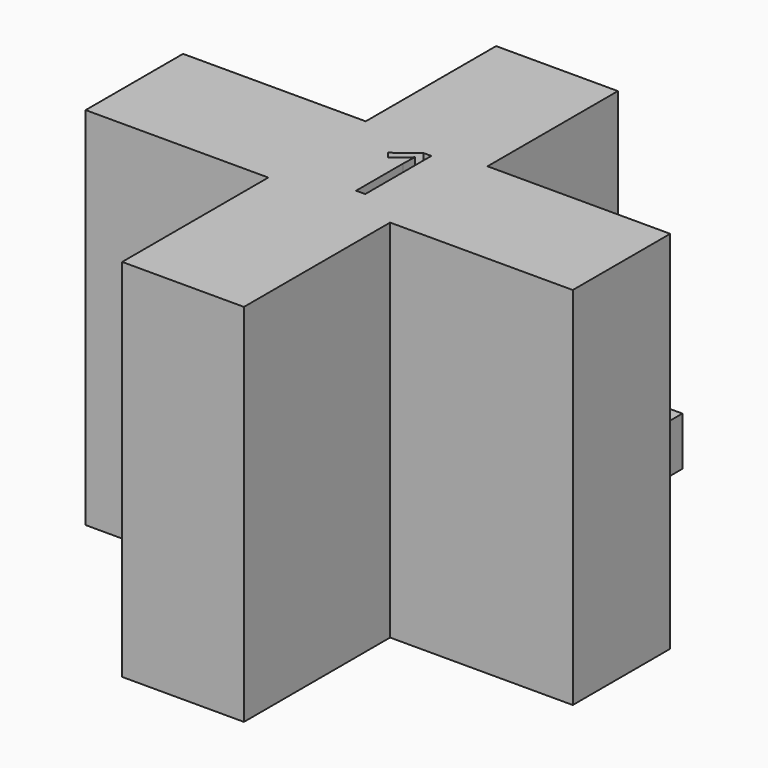
from build123d import *

# Parameters (mm, degrees)
F0_W         = 12.7
F0_H         = 57.15
F1_DEPTH     = 5.08
F2_W         = 50.8
F2_H         = 12.7
F3_DEPTH     = 38.1
F4_W         = 12.7
F4_H         = 48.7413735385
F5_DEPTH     = 33.02
F6_TEXT_SIZE = 12.0747026004
F7_DEPTH     = 2.54


# Not quite as in the source:
# - Text() gives the source's letters only with a copy of the font that has no kerning and outlines rounded to 1/6400 em; it was checked with that copy


with BuildPart() as f1:
    # F0 (on Top) → F1 (new body)
    with BuildSketch(Plane.XY):
        with Locations((-37.0165128261, 2.9978602284)):
            Rectangle(F0_W, F0_H)
    extrude(amount=F1_DEPTH)

    # F2 (on Top) → F3 (join)
    with BuildSketch(Plane.XY):
        with Locations((-37.0165128261, -0.1771397716)):
            Rectangle(F2_W, F2_H)
    extrude(amount=F3_DEPTH)

    # F4 (on face) → F5 (join)
    with BuildSketch(Plane.XY.offset(5.08)):
        with Locations((-37.0165128261, -1.2064530024)):
            Rectangle(F4_W, F4_H)
    extrude(amount=F5_DEPTH)

    # F6 (on face) → F7 (cut)
    with BuildSketch(Plane.XY.offset(38.1)):
        with Locations((-39.5974777639, -3.8714513648)):
            Text('1', F6_TEXT_SIZE, font='Open Sans', text_align=(TextAlign.LEFT, TextAlign.BOTTOM))
    extrude(amount=-F7_DEPTH, mode=Mode.SUBTRACT)


solid = f1.part
